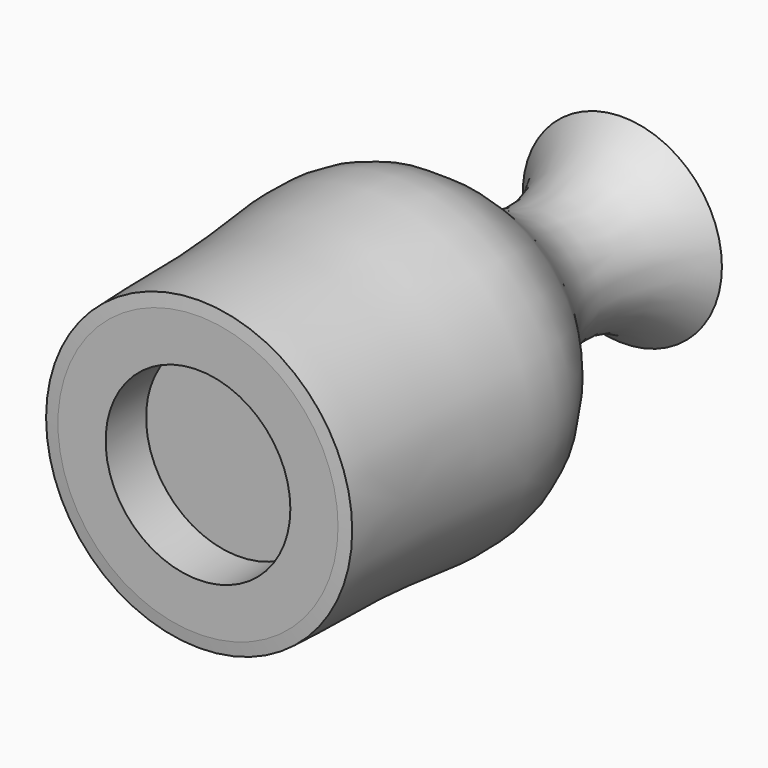
from build123d import *

# Parameters (mm, degrees)
F2_T = 2.5


# Not quite as in the source:
# - a shell that OpenCascade refuses in one call is made with other operations: the cavity is built on its own and cut out


with BuildPart() as f1:
    # F0 (on Top) → F1 (revolve)
    with BuildSketch(Plane.XY):
        with BuildLine():
            Line((17.2804780304, 39.4352339208), (0, 39.4352339208))
            Line((0, 39.4352339208), (0, -43.8134409487))
            Line((0, -43.8134409487), (16.0267315805, -43.8134409487))
            Line((16.0267315805, -43.8134409487), (16.0267315805, -52.5896549225))
            Line((16.0267315805, -52.5896549225), (24.3014525622, -52.5896549225))
            Line((24.3014525622, -52.5896549225), (26.5581905842, -52.3389056325))
            add(Edge.make_bspline(
                [(17.2804780304, 39.4352339208), (15.4241225487, 37.4611710574), (11.1918862105, 32.8213707524), (7.9742124467, 14.100491533), (31.589105581, -1.866812475), (26.1954888157, -27.7072783001), (26.9938640556, -43.9876284398), (26.5581905842, -52.3389056325)],
                knots=[0, 0, 0, 0, 0.1346971319, 0.3184425297, 0.5464554161, 0.7703226354, 1, 1, 1, 1], degree=3))
        make_face()
    revolve(axis=Axis((0, -2.189103514, 0), (0, -1, 0)))

    # F2: shell of thickness 2.5, made by hand


with BuildPart() as f2_core1:
    # F2_t2: copy of F1
    add(f1.part)

    # the walls: a layer under each face that stays
    f2_faces = [f2_core1.faces().sort_by_distance(p)[0] for p in [
        (0, -43.8134409487, 0),
        (-16.0267315805, -48.2015479356, 0),
        (16.2009683748, -52.5896549225, -16.2009683748),
        (-25.4298215732, -52.4642802775, 0),
        (-23.9936965882, 0.7966822698, 0),
    ]]
    thicken(f2_faces, amount=-F2_T, mode=Mode.SUBTRACT)

    # F2_s3 → F2_t4 (revolve, cut)
    with BuildSketch(Plane.XY):
        Polygon((16.0017315805, -43.8384409487), (16.0267315805, -41.3134409487), (18.5267315805, -41.3134409487), (18.5267315805, -43.8134409487), align=None)
    revolve(axis=Axis((0, -43.8134409487, 0), (0, -1, 0)), mode=Mode.SUBTRACT)


with BuildPart() as f1_1:
    add(f1.part)

    # what is left inside the walls is the cavity
    f2_cavity = [f2_core1.part.solids().sort_by_distance(p)[0] for p in [
        (-11.283337, 12.053715, 0),
    ]]
    add(f2_cavity, mode=Mode.SUBTRACT)


solid = f1_1.part
